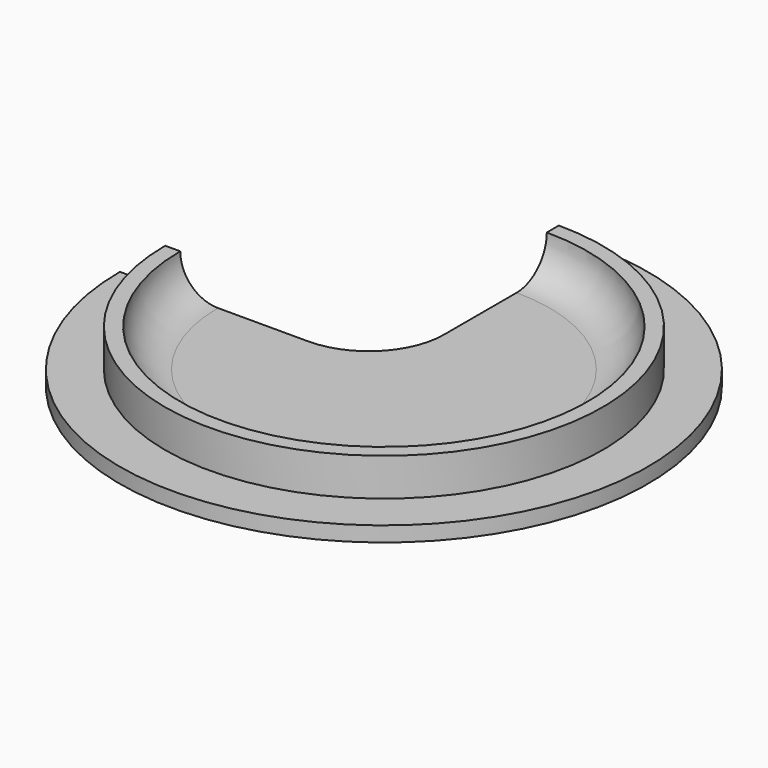
from build123d import *

# Parameters (mm, degrees)
F0_R          = 35
F1_DEPTH      = 2
F2_R          = 29
F3_DEPTH      = 5
F4_R          = 27
F5_DEPTH      = 5
F6_W          = 45.179169625
F6_H          = 45.1430678368
F7_DEPTH      = 2.001
F7_DEPTH_BACK = 5.001
F8_R          = 4.99999
F9_R          = 10


# Not quite as in the source:
# - a fillet or chamfer is up to 0.001 mm smaller than in the source, because OpenCascade refuses the exact size


with BuildPart() as f1:
    # F0 (on Top) → F1 (new body)
    with BuildSketch(Plane.XY):
        Circle(F0_R)
    extrude(amount=F1_DEPTH)

    # F2 (on face) → F3 (join)
    with BuildSketch(Plane.XY.offset(2)):
        Circle(F2_R)
    extrude(amount=F3_DEPTH)

    # F4 (on face) → F5 (cut, through all)
    with BuildSketch(Plane.XY.offset(7)):
        Circle(F4_R)
    extrude(amount=-F5_DEPTH, mode=Mode.SUBTRACT)

    # F6 (on face) → F7 (cut, two sides)
    with BuildSketch(Plane.XY.offset(2)) as f7_sk:
        with Locations((-22.5895848125, 22.5715339184)):
            Rectangle(F6_W, F6_H)
    extrude(amount=-F7_DEPTH, mode=Mode.SUBTRACT)
    extrude(f7_sk.sketch, amount=F7_DEPTH_BACK, mode=Mode.SUBTRACT)

    # F8 (radius 5 in the source; OpenCascade refuses exactly that, so slightly less here)
    f8_edges = [f1.edges().sort_by_distance(p)[0] for p in [
        (19.091883, -19.091883, 2),
    ]]
    fillet(f8_edges, radius=F8_R)

    # F9
    f9_edges = [f1.edges().sort_by_distance(p)[0] for p in [
        (0, 0, 1),
    ]]
    fillet(f9_edges, radius=F9_R)


solid = f1.part
